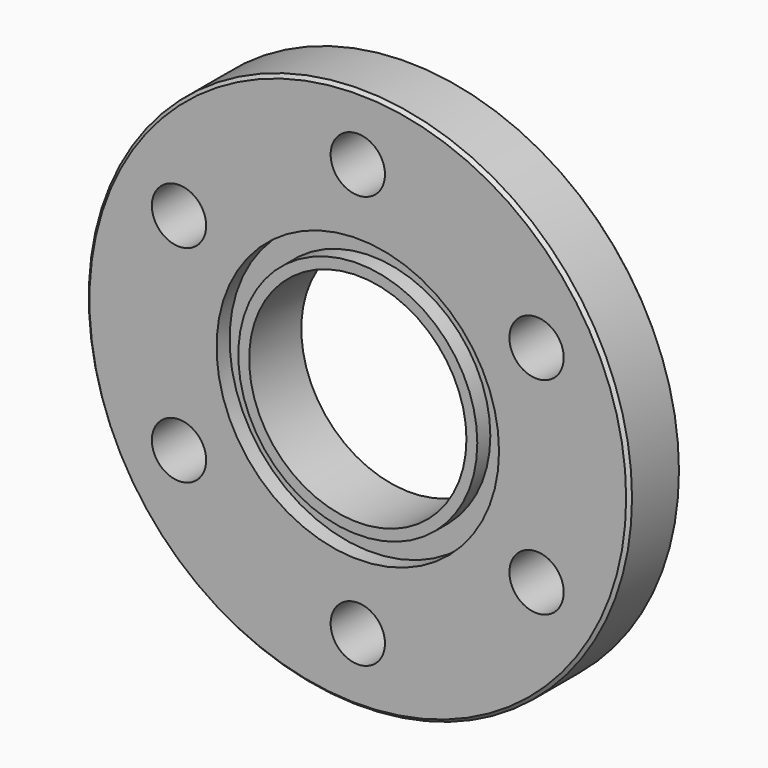
from build123d import *

# Parameters (mm, degrees)
F0_R     = 50
F0_R_2   = 5
F0_R_3   = 26
F0_R_4   = 22
F0_R_5   = 20
F1_DEPTH = 6
F2_R     = 26
F2_R_2   = 22
F3_DEPTH = 3
F5_R     = 26
F5_R_2   = 22
F6_DEPTH = 3
F7_SIZE  = 0.6


with BuildPart() as f1:
    # F0 (on Front) → F1 (new body, symmetric)
    with BuildSketch(Plane.XZ):
        Circle(F0_R)
        with Locations((-32.9089653438, -19)):
            Circle(F0_R_2, mode=Mode.SUBTRACT)
        with Locations((0, -38)):
            Circle(F0_R_2, mode=Mode.SUBTRACT)
        with Locations((32.9089653438, -19)):
            Circle(F0_R_2, mode=Mode.SUBTRACT)
        with Locations((-32.9089653438, 19)):
            Circle(F0_R_2, mode=Mode.SUBTRACT)
        Circle(F0_R_3, mode=Mode.SUBTRACT)
        with Locations((32.9089653438, 19)):
            Circle(F0_R_2, mode=Mode.SUBTRACT)
        with Locations((0, 38)):
            Circle(F0_R_2, mode=Mode.SUBTRACT)
        Circle(F0_R_3)
        Circle(F0_R_4, mode=Mode.SUBTRACT)
        Circle(F0_R_4)
        Circle(F0_R_5, mode=Mode.SUBTRACT)
    extrude(amount=F1_DEPTH, both=True)

    # F2 (on face) → F3 (cut)
    with BuildSketch(Plane.XZ.offset(6)):
        Circle(F2_R)
        Circle(F2_R_2, mode=Mode.SUBTRACT)
    extrude(amount=-F3_DEPTH, mode=Mode.SUBTRACT)

    # F5 (on face) → F6 (cut)
    with BuildSketch(Plane(origin=(0, 6, 0), x_dir=(-1, 0, 0), z_dir=(0, 1, 0))):
        Circle(F5_R)
        Circle(F5_R_2, mode=Mode.SUBTRACT)
    extrude(amount=-F6_DEPTH, mode=Mode.SUBTRACT)

    # F7
    f7_edges = [f1.edges().sort_by_distance(p)[0] for p in [
        (-50, 6, 0),
        (50, 0, 0),
        (-50, -6, 0),
    ]]
    chamfer(f7_edges, length=F7_SIZE)


solid = f1.part
